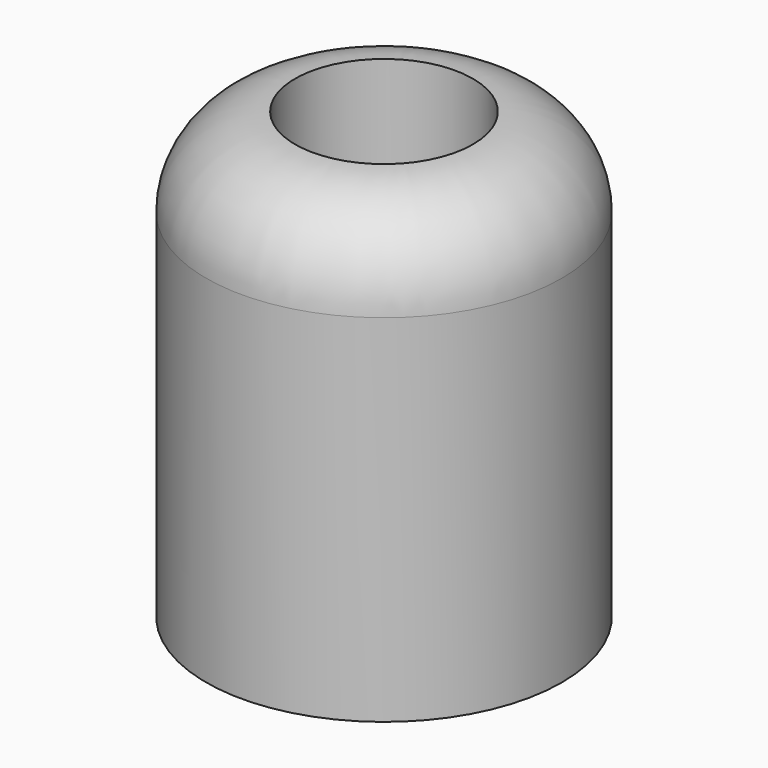
from build123d import *

# Parameters (mm, degrees)
F0_R     = 10
F0_R_2   = 5
F1_DEPTH = 25
F2_DEPTH = 25
F3_R     = 4.99999


# Not quite as in the source:
# - a fillet or chamfer is up to 0.001 mm smaller than in the source, because OpenCascade refuses the exact size


with BuildPart() as f1:
    # F0 (on Top) → F1 (new body)
    with BuildSketch(Plane.XY):
        Circle(F0_R)
        Circle(F0_R_2, mode=Mode.SUBTRACT)
    extrude(amount=F1_DEPTH)

    # F0 (on Top) → F2 (join)
    with BuildSketch(Plane.XY):
        Circle(F0_R)
        Circle(F0_R_2, mode=Mode.SUBTRACT)
    extrude(amount=F2_DEPTH)

    # F3 (radius 5 in the source; OpenCascade refuses exactly that, so slightly less here)
    f3_edges = [f1.edges().sort_by_distance(p)[0] for p in [
        (-10, 0, 25),
    ]]
    fillet(f3_edges, radius=F3_R)


solid = f1.part
